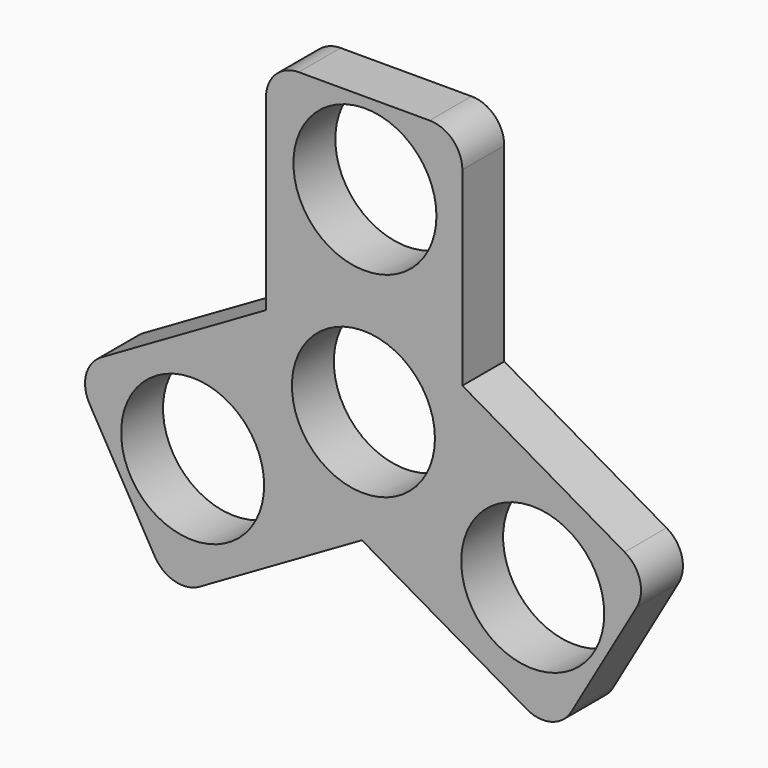
from build123d import *

# Parameters (mm, degrees)
F0_R     = 10.925
F1_DEPTH = 8


with BuildPart() as f1:
    # F0 (on Front) → F1 (new body)
    with BuildSketch(Plane.XZ):
        with BuildLine():
            Line((-136.3183801476, -4.150791151), (-136.3183801476, -8.1894561753))
            Line((-136.3183801476, -8.1894561753), (-143.3135531644, -8.1894561753))
            Line((-143.3135531644, -8.1894561753), (-151.6621599046, -13.0095265241))
            Line((-151.6621599046, -13.0095265241), (-126.5146964668, -27.5284213094))
            ThreePointArc((-126.5146964668, -27.5284213094), (-122.7206012413, -28.027923422), (-119.6845694479, -25.6982942905))
            Line((-119.6845694479, -25.6982942905), (-109.6845694479, -8.3777862148))
            ThreePointArc((-109.6845694479, -8.3777862148), (-109.1850673353, -4.5836909893), (-111.5146964668, -1.5476591959))
            Line((-111.5146964668, -1.5476591959), (-136.3183801476, 12.7727542541))
            Line((-136.3183801476, 12.7727542541), (-136.3183801476, 3.1326135564))
            Line((-136.3183801476, 3.1326135564), (-133.1645733963, -2.3299399742))
            Line((-133.1645733963, -2.3299399742), (-136.3183801476, -4.150791151))
        make_face()
        with Locations((-125.5675627039, -10.8870620569)):
            Circle(F0_R, mode=Mode.SUBTRACT)
        Polygon((-144.6669868879, 17.592824603), (-136.3183801476, 3.1326135564), (-136.3183801476, 12.7727542541), align=None)
        Polygon((-157.9697734074, 17.9897872735), (-151.6621599046, 21.6314896272), (-154.815966656, 23.4523408041), align=None)
        with BuildLine():
            Line((-144.6669868879, 17.592824603), (-136.3183801476, 12.7727542541))
            Line((-136.3183801476, 12.7727542541), (-136.3183801476, 41.8105438247))
            ThreePointArc((-136.3183801476, 41.8105438247), (-137.7828462417, 45.3460777306), (-141.3183801476, 46.8105438247))
            Line((-141.3183801476, 46.8105438247), (-161.3183801476, 46.8105438247))
            ThreePointArc((-161.3183801476, 46.8105438247), (-164.8539140536, 45.3460777306), (-166.3183801476, 41.8105438247))
            Line((-166.3183801476, 41.8105438247), (-166.3183801476, 13.1697169246))
            Line((-166.3183801476, 13.1697169246), (-157.9697734074, 17.9897872735))
            Line((-157.9697734074, 17.9897872735), (-154.815966656, 23.4523408041))
            Line((-154.815966656, 23.4523408041), (-151.6621599046, 21.6314896272))
            Line((-151.6621599046, 21.6314896272), (-148.1645733963, 23.6508221394))
            Line((-148.1645733963, 23.6508221394), (-144.6669868879, 17.592824603))
        make_face()
        with Locations((-151.2037868953, 34.3101060979)):
            Circle(F0_R, mode=Mode.SUBTRACT)
        Polygon((-166.3183801476, 13.1697169246), (-166.3183801476, 3.5295762269), (-157.9697734074, 17.9897872735), align=None)
        with BuildLine():
            Line((-151.6621599046, -13.0095265241), (-160.0107666449, -8.1894561753))
            Line((-160.0107666449, -8.1894561753), (-166.3183801476, -8.1894561753))
            Line((-166.3183801476, -8.1894561753), (-166.3183801476, -4.5477538216))
            Line((-166.3183801476, -4.5477538216), (-169.815966656, -2.5284213094))
            Line((-169.815966656, -2.5284213094), (-166.3183801476, 3.5295762269))
            Line((-166.3183801476, 3.5295762269), (-166.3183801476, 13.1697169246))
            Line((-166.3183801476, 13.1697169246), (-191.4658435855, -1.3491778606))
            ThreePointArc((-191.4658435855, -1.3491778606), (-193.7954727169, -4.3852096541), (-193.2959706044, -8.1793048796))
            Line((-193.2959706044, -8.1793048796), (-183.2959706044, -25.4998129553))
            ThreePointArc((-183.2959706044, -25.4998129553), (-180.259938811, -27.8294420867), (-176.4658435855, -27.3299399742))
            Line((-176.4658435855, -27.3299399742), (-151.6621599046, -13.0095265241))
        make_face()
        with Locations((-177.5275706007, -10.4900993864)):
            Circle(F0_R, mode=Mode.SUBTRACT)
        Polygon((-160.0107666449, -8.1894561753), (-143.3135531644, -8.1894561753), (-136.3183801476, -4.150791151), (-136.3183801476, 3.1326135564), (-144.6669868879, 17.592824603), (-151.6621599046, 21.6314896272), (-157.9697734074, 17.9897872735), (-166.3183801476, 3.5295762269), (-166.3183801476, -4.5477538216), align=None)
        with Locations((-151.4329734, 4.3109815515)):
            Circle(F0_R, mode=Mode.SUBTRACT)
        Polygon((-169.815966656, -2.5284213094), (-166.3183801476, -4.5477538216), (-166.3183801476, 3.5295762269), align=None)
        Polygon((-151.6621599046, 21.6314896272), (-144.6669868879, 17.592824603), (-148.1645733963, 23.6508221394), align=None)
        Polygon((-136.3183801476, 3.1326135564), (-136.3183801476, -4.150791151), (-133.1645733963, -2.3299399742), align=None)
        Polygon((-143.3135531644, -8.1894561753), (-136.3183801476, -8.1894561753), (-136.3183801476, -4.150791151), align=None)
        Polygon((-166.3183801476, -8.1894561753), (-160.0107666449, -8.1894561753), (-166.3183801476, -4.5477538216), align=None)
        Polygon((-151.6621599046, -13.0095265241), (-143.3135531644, -8.1894561753), (-160.0107666449, -8.1894561753), align=None)
    extrude(amount=F1_DEPTH)


solid = f1.part
